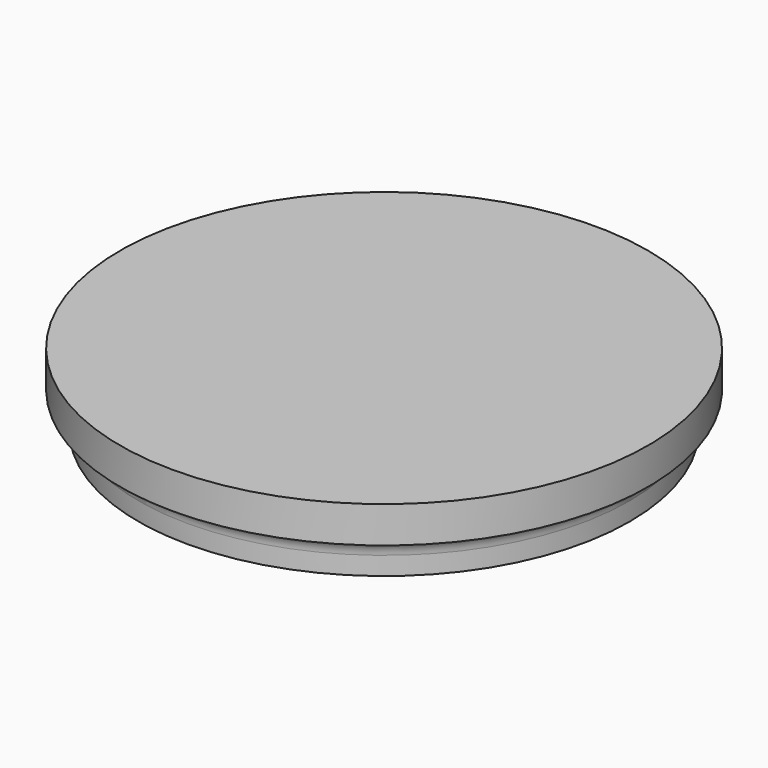
from build123d import *

# Parameters (mm, degrees)
F0_W   = 25
F0_H   = 2
F0_W_2 = 2
F0_H_2 = 4
F2_R   = 1.99999


# Not quite as in the source:
# - a fillet or chamfer is up to 0.001 mm smaller than in the source, because OpenCascade refuses the exact size


with BuildPart() as f1:
    # F0 (on Right) → F1 (revolve)
    with BuildSketch(Plane.YZ):
        with Locations((-12.5, -1)):
            Rectangle(F0_W, F0_H)
        Polygon((-27, -4), (-25, -4), (-25, -2), (-25, 0), (-29, 0), (-29, -4), align=None)
        with Locations((-26, -6)):
            Rectangle(F0_W_2, F0_H_2)
    revolve(axis=Axis((0, 0, -1), (0, 0, -1)))

    # F2 (radius 2 in the source; OpenCascade refuses exactly that, so slightly less here)
    f2_edges = [f1.edges().sort_by_distance(p)[0] for p in [
        (0, 27, -4),
    ]]
    fillet(f2_edges, radius=F2_R)


solid = f1.part
